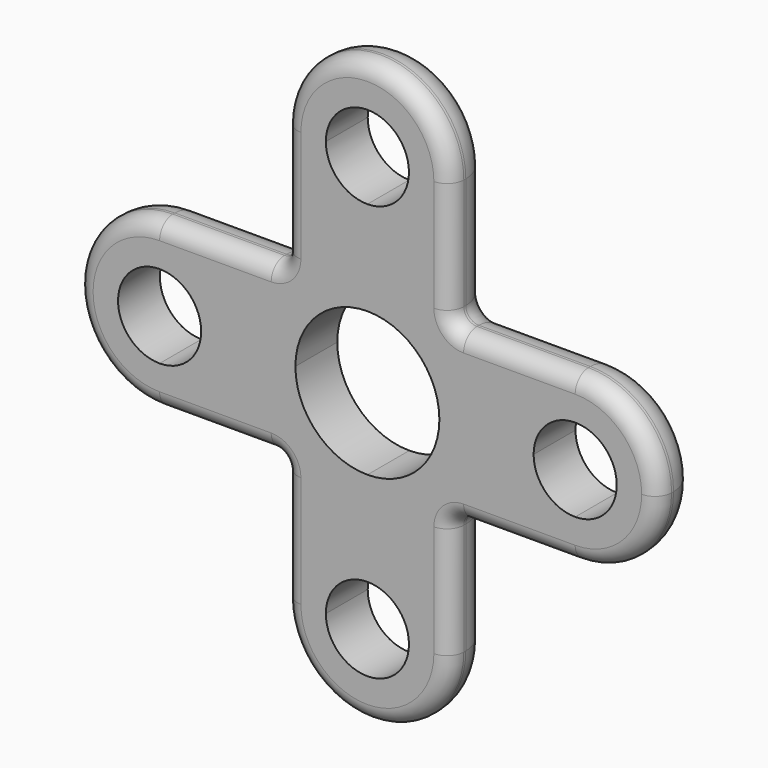
from build123d import *

# Parameters (mm, degrees)
F1_DEPTH = 4
F2_R     = 2
F3_R     = 5.08
F4_R     = 2.54


with BuildPart() as f1:
    # F0 (on Front) → F1 (new body, symmetric)
    with BuildSketch(Plane.XZ):
        with BuildLine():
            ThreePointArc((-19.05, 0), (-22.769744, -8.980256), (-31.75, -12.7))
            Line((-31.75, -12.7), (-12.7, -12.7))
            Line((-12.7, -12.7), (-12.7, 0))
            Line((-12.7, 0), (-19.05, 0))
        make_face()
        with BuildLine():
            ThreePointArc((-31.75, 12.7), (-44.45, 0), (-31.75, -12.7))
            Line((-31.75, -12.7), (-31.75, -6.35))
            ThreePointArc((-31.75, -6.35), (-38.1, 0), (-31.75, 6.35))
            Line((-31.75, 6.35), (-31.75, 12.7))
        make_face()
        with BuildLine():
            Line((-31.75, -6.35), (-31.75, -12.7))
            ThreePointArc((-31.75, -12.7), (-22.769744, -8.980256), (-19.05, 0))
            Line((-19.05, 0), (-25.4, 0))
            ThreePointArc((-25.4, 0), (-27.259872, -4.490128), (-31.75, -6.35))
        make_face()
        with BuildLine():
            Line((-12.7, 0), (-12.7, -12.7))
            Line((-12.7, -12.7), (0, -12.7))
            Line((0, -12.7), (0, -11))
            ThreePointArc((0, -11), (-7.778175, -7.778175), (-11, 0))
            Line((-11, 0), (-12.7, 0))
        make_face()
        with BuildLine():
            Line((0, -12.7), (-12.7, -12.7))
            Line((-12.7, -12.7), (-12.7, -31.75))
            ThreePointArc((-12.7, -31.75), (-8.980256, -22.769744), (0, -19.05))
            Line((0, -19.05), (0, -12.7))
        make_face()
        with BuildLine():
            ThreePointArc((-19.05, 0), (-22.769744, 8.980256), (-31.75, 12.7))
            Line((-31.75, 12.7), (-31.75, 6.35))
            ThreePointArc((-31.75, 6.35), (-27.259872, 4.490128), (-25.4, 0))
            Line((-25.4, 0), (-19.05, 0))
        make_face()
        with BuildLine():
            Line((-12.7, 12.7), (-31.75, 12.7))
            ThreePointArc((-31.75, 12.7), (-22.769744, 8.980256), (-19.05, 0))
            Line((-19.05, 0), (-12.7, 0))
            Line((-12.7, 0), (-12.7, 12.7))
        make_face()
        with BuildLine():
            Line((0, -11), (0, -12.7))
            Line((0, -12.7), (12.7, -12.7))
            Line((12.7, -12.7), (12.7, 0))
            Line((12.7, 0), (11, 0))
            ThreePointArc((11, 0), (7.778175, -7.778175), (0, -11))
        make_face()
        with BuildLine():
            Line((12.7, -12.7), (0, -12.7))
            Line((0, -12.7), (0, -19.05))
            ThreePointArc((0, -19.05), (8.980256, -22.769744), (12.7, -31.75))
            Line((12.7, -31.75), (12.7, -12.7))
        make_face()
        with BuildLine():
            Line((-12.7, 12.7), (-12.7, 0))
            Line((-12.7, 0), (-11, 0))
            ThreePointArc((-11, 0), (-7.778175, 7.778175), (0, 11))
            Line((0, 11), (0, 12.7))
            Line((0, 12.7), (-12.7, 12.7))
        make_face()
        with BuildLine():
            ThreePointArc((0, -19.05), (-8.980256, -22.769744), (-12.7, -31.75))
            Line((-12.7, -31.75), (-6.35, -31.75))
            ThreePointArc((-6.35, -31.75), (-4.490128, -27.259872), (0, -25.4))
            Line((0, -25.4), (0, -19.05))
        make_face()
        with BuildLine():
            Line((-6.35, -31.75), (-12.7, -31.75))
            ThreePointArc((-12.7, -31.75), (0, -44.45), (12.7, -31.75))
            Line((12.7, -31.75), (6.35, -31.75))
            ThreePointArc((6.35, -31.75), (0, -38.1), (-6.35, -31.75))
        make_face()
        with BuildLine():
            Line((-12.7, 31.75), (-12.7, 12.7))
            Line((-12.7, 12.7), (0, 12.7))
            Line((0, 12.7), (0, 19.05))
            ThreePointArc((0, 19.05), (-8.980256, 22.769744), (-12.7, 31.75))
        make_face()
        with BuildLine():
            Line((12.7, 0), (12.7, -12.7))
            Line((12.7, -12.7), (31.75, -12.7))
            ThreePointArc((31.75, -12.7), (22.769744, -8.980256), (19.05, 0))
            Line((19.05, 0), (12.7, 0))
        make_face()
        with BuildLine():
            ThreePointArc((12.7, -31.75), (8.980256, -22.769744), (0, -19.05))
            Line((0, -19.05), (0, -25.4))
            ThreePointArc((0, -25.4), (4.490128, -27.259872), (6.35, -31.75))
            Line((6.35, -31.75), (12.7, -31.75))
        make_face()
        with BuildLine():
            Line((0, 19.05), (0, 12.7))
            Line((0, 12.7), (12.7, 12.7))
            Line((12.7, 12.7), (12.7, 31.75))
            ThreePointArc((12.7, 31.75), (8.980256, 22.769744), (0, 19.05))
        make_face()
        with BuildLine():
            Line((12.7, 12.7), (0, 12.7))
            Line((0, 12.7), (0, 11))
            ThreePointArc((0, 11), (7.778175, 7.778175), (11, 0))
            Line((11, 0), (12.7, 0))
            Line((12.7, 0), (12.7, 12.7))
        make_face()
        with BuildLine():
            ThreePointArc((12.7, 31.75), (0, 44.45), (-12.7, 31.75))
            Line((-12.7, 31.75), (-6.35, 31.75))
            ThreePointArc((-6.35, 31.75), (0, 38.1), (6.35, 31.75))
            Line((6.35, 31.75), (12.7, 31.75))
        make_face()
        with BuildLine():
            Line((-6.35, 31.75), (-12.7, 31.75))
            ThreePointArc((-12.7, 31.75), (-8.980256, 22.769744), (0, 19.05))
            Line((0, 19.05), (0, 25.4))
            ThreePointArc((0, 25.4), (-4.490128, 27.259872), (-6.35, 31.75))
        make_face()
        with BuildLine():
            ThreePointArc((19.05, 0), (22.769744, -8.980256), (31.75, -12.7))
            Line((31.75, -12.7), (31.75, -6.35))
            ThreePointArc((31.75, -6.35), (27.259872, -4.490128), (25.4, 0))
            Line((25.4, 0), (19.05, 0))
        make_face()
        with BuildLine():
            Line((31.75, -6.35), (31.75, -12.7))
            ThreePointArc((31.75, -12.7), (40.730256, -8.980256), (44.45, 0))
            ThreePointArc((44.45, 0), (40.730256, 8.980256), (31.75, 12.7))
            Line((31.75, 12.7), (31.75, 6.35))
            ThreePointArc((31.75, 6.35), (36.240128, 4.490128), (38.1, 0))
            ThreePointArc((38.1, 0), (36.240128, -4.490128), (31.75, -6.35))
        make_face()
        with BuildLine():
            Line((12.7, 12.7), (12.7, 0))
            Line((12.7, 0), (19.05, 0))
            ThreePointArc((19.05, 0), (22.769744, 8.980256), (31.75, 12.7))
            Line((31.75, 12.7), (12.7, 12.7))
        make_face()
        with BuildLine():
            Line((0, 25.4), (0, 19.05))
            ThreePointArc((0, 19.05), (8.980256, 22.769744), (12.7, 31.75))
            Line((12.7, 31.75), (6.35, 31.75))
            ThreePointArc((6.35, 31.75), (4.490128, 27.259872), (0, 25.4))
        make_face()
        with BuildLine():
            ThreePointArc((31.75, 12.7), (22.769744, 8.980256), (19.05, 0))
            Line((19.05, 0), (25.4, 0))
            ThreePointArc((25.4, 0), (27.259872, 4.490128), (31.75, 6.35))
            Line((31.75, 6.35), (31.75, 12.7))
        make_face()
    extrude(amount=F1_DEPTH, both=True)

    # F2
    f2_edges = [f1.edges().sort_by_distance(p)[0] for p in [
        (12.7, 0, 12.7),
        (12.7, 0, -12.7),
        (-12.7, 0, -12.7),
        (-12.7, 0, 12.7),
    ]]
    fillet(f2_edges, radius=F2_R)

    # F3
    f3_edges = [f1.edges().sort_by_distance(p)[0] for p in [
        (23.225, 4, 12.7),
    ]]
    fillet(f3_edges, radius=F3_R)

    # F4
    f4_edges = [f1.edges().sort_by_distance(p)[0] for p in [
        (12.7, -4, 23.225),
    ]]
    fillet(f4_edges, radius=F4_R)


solid = f1.part
